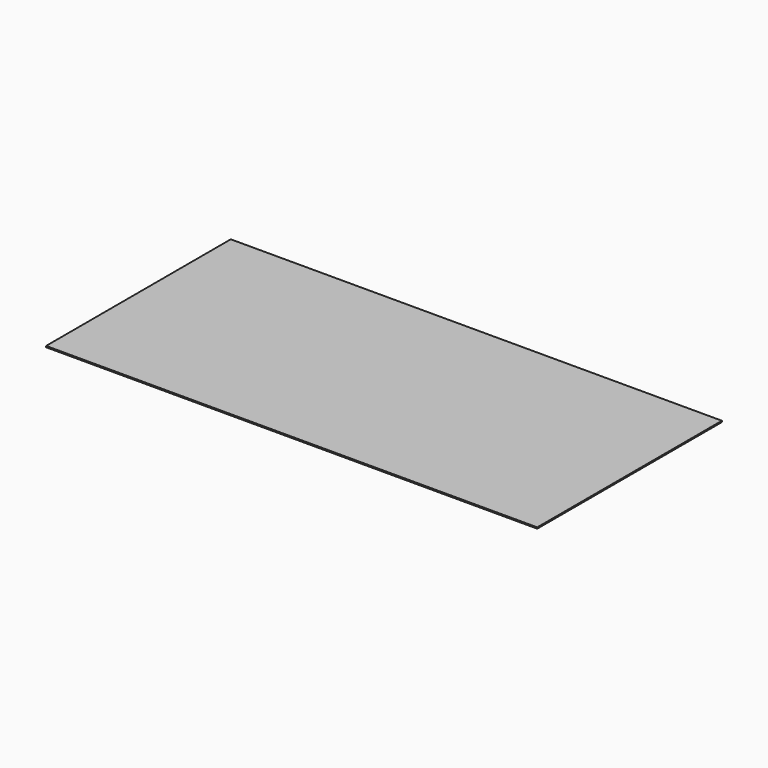
from build123d import *

# Parameters (mm, degrees)
F0_W     = 317.5
F0_H     = 149.225
F1_DEPTH = 0.79375


# Not quite as in the source:
# - a length typed as a fraction of an inch, garbled in the dataset ("3 / 203.2 mm" for 3/8 in), is restored


with BuildPart() as f1:
    # F0 (on Top) → F1 (new body)
    with BuildSketch(Plane.XY):
        Rectangle(F0_W, F0_H)
    extrude(amount=F1_DEPTH)


solid = f1.part
